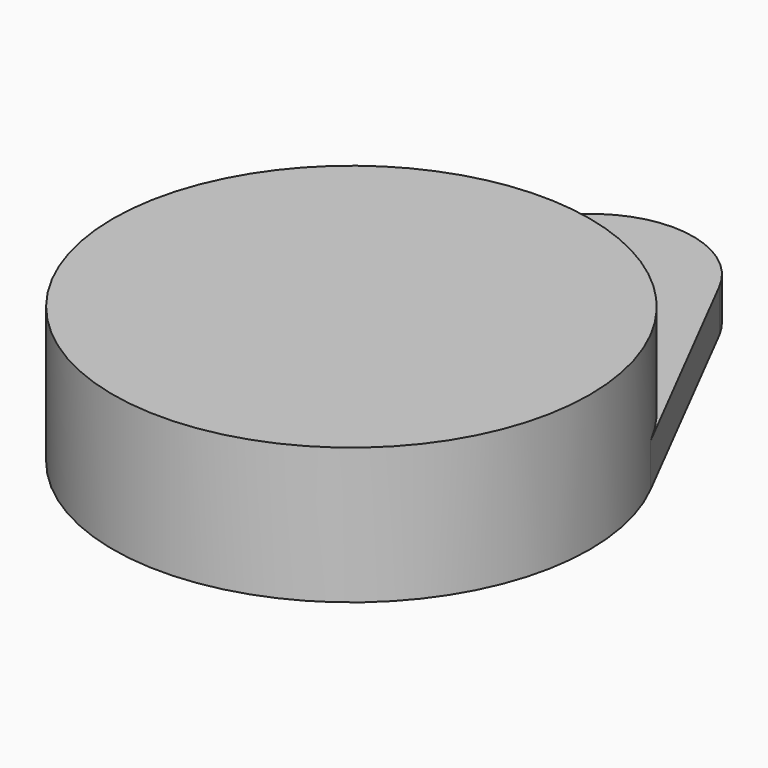
from build123d import *

# Parameters (mm, degrees)
F0_R     = 3.81
F1_DEPTH = 4
F2_DEPTH = 12.7
F3_DEPTH = 10


# Not quite as in the source:
# - a feature names something its author has since deleted; it is built from what else it names


with BuildPart() as f1:
    # F0 (on Top) → F1 (new body)
    with BuildSketch(Plane.XY):
        with BuildLine():
            ThreePointArc((6.7162400934, 21.1859090909), (14.3680496868, 16.9561131513), (19.7963307394, 10.1022727273))
            Line((19.7963307394, 10.1022727273), (8.4841417455, 32.2695454545))
            ThreePointArc((8.4841417455, 32.2695454545), (9.2611304689, 30.1664517595), (9.525, 27.94))
            ThreePointArc((9.525, 27.94), (8.7948226784, 24.2825802736), (6.7162400934, 21.1859090909))
        make_face()
        with BuildLine():
            Line((-8.4841417455, 32.2695454545), (-19.7963307394, 10.1022727273))
            ThreePointArc((-19.7963307394, 10.1022727273), (-14.3680496868, 16.9561131513), (-6.7162400934, 21.1859090909))
            ThreePointArc((-6.7162400934, 21.1859090909), (-9.4060964683, 26.4396752924), (-8.4841417455, 32.2695454545))
        make_face()
        with BuildLine():
            ThreePointArc((-19.7963307394, 10.1022727273), (-5.1950541054, -21.6093044275), (22.225, 0))
            ThreePointArc((22.225, 0), (21.6093044275, 5.1950541054), (19.7963307394, 10.1022727273))
            ThreePointArc((19.7963307394, 10.1022727273), (14.3680496868, 16.9561131513), (6.7162400934, 21.1859090909))
            ThreePointArc((6.7162400934, 21.1859090909), (0, 18.415), (-6.7162400934, 21.1859090909))
            ThreePointArc((-6.7162400934, 21.1859090909), (-14.3680496868, 16.9561131513), (-19.7963307394, 10.1022727273))
        make_face()
        with BuildLine():
            ThreePointArc((-6.7162400934, 21.1859090909), (0, 22.225), (6.7162400934, 21.1859090909))
            ThreePointArc((6.7162400934, 21.1859090909), (8.7948226784, 24.2825802736), (9.525, 27.94))
            ThreePointArc((9.525, 27.94), (9.2611304689, 30.1664517595), (8.4841417455, 32.2695454545))
            ThreePointArc((8.4841417455, 32.2695454545), (0, 37.465), (-8.4841417455, 32.2695454545))
            ThreePointArc((-8.4841417455, 32.2695454545), (-9.4060964683, 26.4396752924), (-6.7162400934, 21.1859090909))
        make_face()
        with Locations((0, 27.94)):
            Circle(F0_R, mode=Mode.SUBTRACT)
        with BuildLine():
            ThreePointArc((-6.7162400934, 21.1859090909), (0, 18.415), (6.7162400934, 21.1859090909))
            ThreePointArc((6.7162400934, 21.1859090909), (0, 22.225), (-6.7162400934, 21.1859090909))
        make_face()
    extrude(amount=F1_DEPTH)

    # F0 (on Top) → F2 (join)
    with BuildSketch(Plane.XY):
        with BuildLine():
            ThreePointArc((-19.7963307394, 10.1022727273), (-5.1950541054, -21.6093044275), (22.225, 0))
            ThreePointArc((22.225, 0), (21.6093044275, 5.1950541054), (19.7963307394, 10.1022727273))
            ThreePointArc((19.7963307394, 10.1022727273), (14.3680496868, 16.9561131513), (6.7162400934, 21.1859090909))
            ThreePointArc((6.7162400934, 21.1859090909), (0, 18.415), (-6.7162400934, 21.1859090909))
            ThreePointArc((-6.7162400934, 21.1859090909), (-14.3680496868, 16.9561131513), (-19.7963307394, 10.1022727273))
        make_face()
        with BuildLine():
            ThreePointArc((-6.7162400934, 21.1859090909), (0, 18.415), (6.7162400934, 21.1859090909))
            ThreePointArc((6.7162400934, 21.1859090909), (0, 22.225), (-6.7162400934, 21.1859090909))
        make_face()
    extrude(amount=F2_DEPTH)

    # F0 (on Top) → F3 (join)
    with BuildSketch(Plane.XY):
        with BuildLine():
            ThreePointArc((-6.7162400934, 21.1859090909), (0, 18.415), (6.7162400934, 21.1859090909))
            ThreePointArc((6.7162400934, 21.1859090909), (0, 22.225), (-6.7162400934, 21.1859090909))
        make_face()
        with BuildLine():
            ThreePointArc((-19.7963307394, 10.1022727273), (-5.1950541054, -21.6093044275), (22.225, 0))
            ThreePointArc((22.225, 0), (21.6093044275, 5.1950541054), (19.7963307394, 10.1022727273))
            ThreePointArc((19.7963307394, 10.1022727273), (14.3680496868, 16.9561131513), (6.7162400934, 21.1859090909))
            ThreePointArc((6.7162400934, 21.1859090909), (0, 18.415), (-6.7162400934, 21.1859090909))
            ThreePointArc((-6.7162400934, 21.1859090909), (-14.3680496868, 16.9561131513), (-19.7963307394, 10.1022727273))
        make_face()
    extrude(amount=F3_DEPTH)


solid = f1.part
